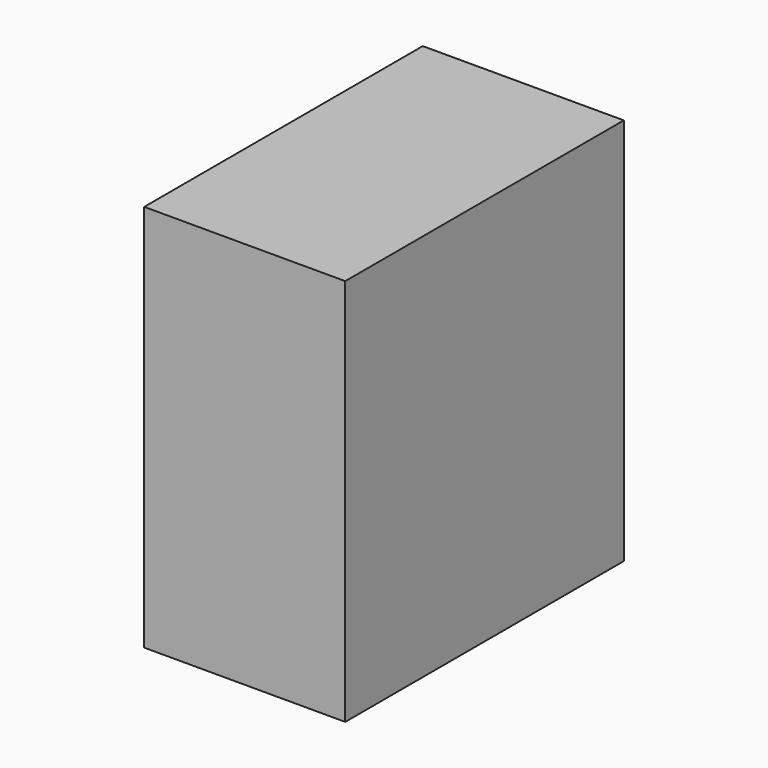
from build123d import *

# Parameters (mm, degrees)
F1_W     = 55.4384309798
F1_H     = 96.0222035646
F2_DEPTH = 25.399999693
F3_DEPTH = 81.6175211221


# Not quite as in the source:
# - a feature names something its author has since deleted; it is built from what else it names


with BuildPart() as f2:
    # F1 (on Top) → F2 (new body)
    with BuildSketch(Plane.XY):
        with Locations((-15.6900202855, -80.130405724)):
            Rectangle(F1_W, F1_H)
    extrude(amount=-F2_DEPTH)

    # F3 (add): a face of the model
    f3_faces = [f2.faces().sort_by_distance(p)[0] for p in [
        (-15.6900202855, -80.130405724, 0),
    ]]
    extrude(f3_faces, amount=F3_DEPTH)


solid = f2.part
